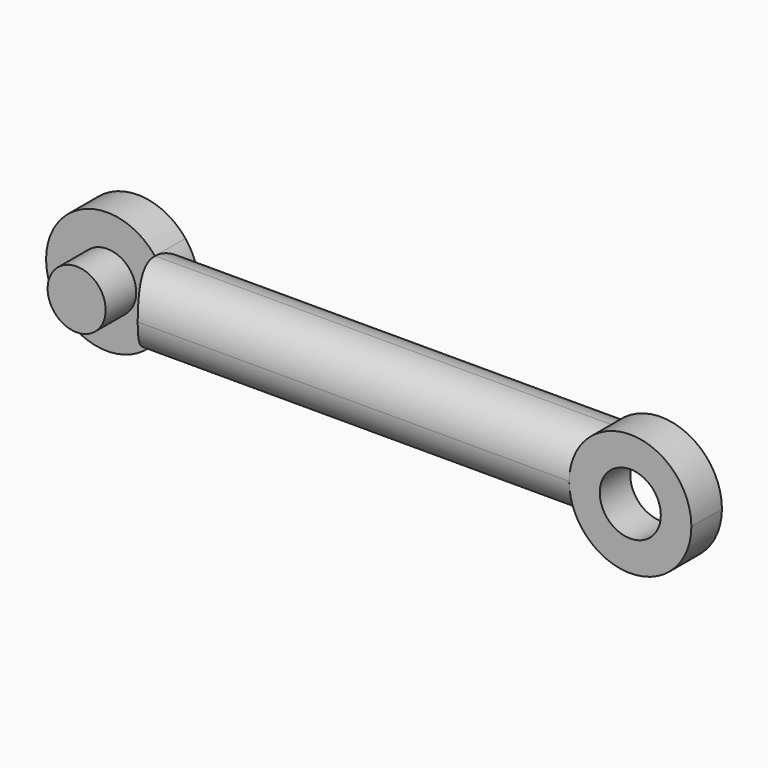
from build123d import *

# Parameters (mm, degrees)
F1_DEPTH = 6.35
F2_R     = 6.3499
F0_R     = 5.08
F3_DEPTH = 6.35
F0_R_2   = 4.826
F4_DEPTH = 6.35
F5_DEPTH = 6.35


# Not quite as in the source:
# - a fillet or chamfer is up to 0.001 mm smaller than in the source, because OpenCascade refuses the exact size


with BuildPart() as f1:
    # F0 (on Front) → F1 (new body, symmetric)
    with BuildSketch(Plane.XZ):
        with BuildLine():
            Line((38.1, 6.35), (-38.1, 6.35))
            ThreePointArc((-38.1, 6.35), (-36.4445407024, 3.3649028089), (-35.871147458, 0))
            ThreePointArc((-35.871147458, 0), (-36.4445407024, -3.3649028089), (-38.1, -6.35))
            Line((-38.1, -6.35), (38.1, -6.35))
            ThreePointArc((38.1, -6.35), (35.871147458, 0), (38.1, 6.35))
        make_face()
    extrude(amount=F1_DEPTH, both=True)

    # F2 (radius 6.35 in the source; OpenCascade refuses exactly that, so slightly less here)
    f2_edges = [f1.edges().sort_by_distance(p)[0] for p in [
        (0, -6.35, 6.35),
        (0, 6.35, 6.35),
        (0, -6.35, -6.35),
        (0, 6.35, -6.35),
    ]]
    fillet(f2_edges, radius=F2_R)

    # F0 (on Front) → F3 (join)
    with BuildSketch(Plane.XZ):
        with BuildLine():
            Line((38.1, -6.35), (38.1, 6.35))
            ThreePointArc((38.1, 6.35), (35.871147458, 0), (38.1, -6.35))
        make_face()
        with BuildLine():
            ThreePointArc((56.191147458, 0), (49.3960502669, 9.5866067556), (38.1, 6.35))
            Line((38.1, 6.35), (38.1, -6.35))
            ThreePointArc((38.1, -6.35), (49.3960502669, -9.5866067556), (56.191147458, 0))
        make_face()
        with Locations((46.031147458, 0)):
            Circle(F0_R, mode=Mode.SUBTRACT)
    extrude(amount=F3_DEPTH)

    # F0 (on Front) → F4 (join)
    with BuildSketch(Plane.XZ):
        with BuildLine():
            Line((-38.1, -6.35), (-38.1, 6.35))
            ThreePointArc((-38.1, 6.35), (-56.191147458, 0), (-38.1, -6.35))
        make_face()
        with Locations((-46.031147458, 0)):
            Circle(F0_R_2, mode=Mode.SUBTRACT)
        with BuildLine():
            ThreePointArc((-35.871147458, 0), (-36.4445407024, 3.3649028089), (-38.1, 6.35))
            Line((-38.1, 6.35), (-38.1, -6.35))
            ThreePointArc((-38.1, -6.35), (-36.4445407024, -3.3649028089), (-35.871147458, 0))
        make_face()
    extrude(amount=-F4_DEPTH)

    # F0 (on Front) → F5 (join, symmetric)
    with BuildSketch(Plane.XZ):
        with Locations((-46.031147458, 0)):
            Circle(F0_R_2)
    extrude(amount=F5_DEPTH, both=True)


solid = f1.part
